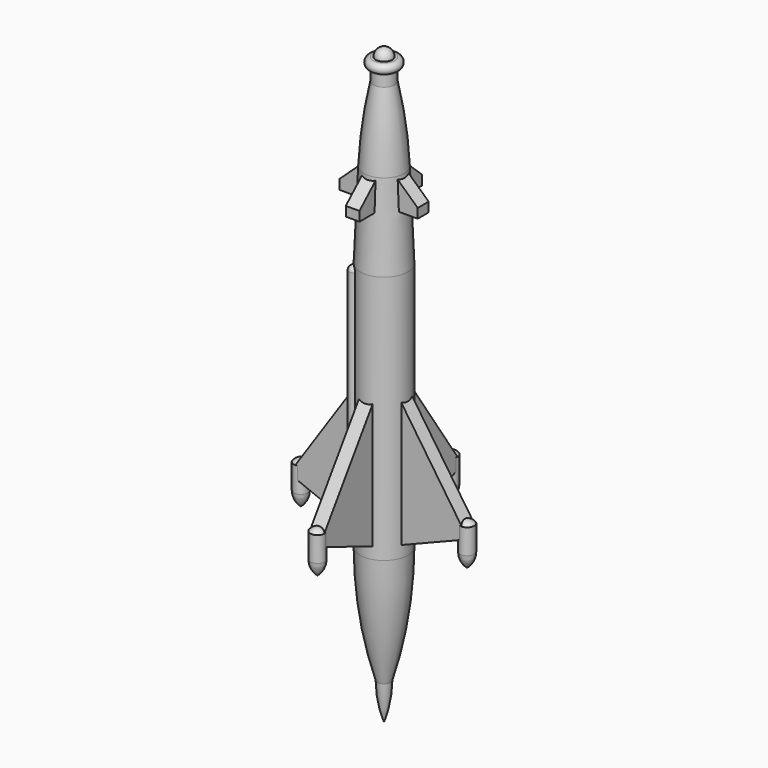
from build123d import *

# Parameters (mm, degrees)
F4_DEPTH     = 0.2
F7_COUNT     = 4
F10_DEPTH    = 6.25
F11_T4_ANGLE = 107.9477893391
F11_S5_R     = 0.1388888889
F11_T6_DEPTH = 2
F12_R        = 0.138879


# Not quite as in the source:
# - a fillet or chamfer that OpenCascade refuses, or shapes differently, is made with other operations: its cross-section is extruded or revolved along the edge and cut away or added
# - a fillet or chamfer is up to 0.001 mm smaller than in the source, because OpenCascade refuses the exact size
# - a feature names something its author has since deleted; it is built from what else it names


with BuildPart() as f2:
    # F1 (on Front) → F2 (revolve)
    with BuildSketch(Plane.XZ):
        with BuildLine():
            Line((0, 17.3611111111), (0, 0))
            ThreePointArc((0, 0), (0.1428592565, 0.5297895315), (0.1909722222, 1.0763888889))
            ThreePointArc((0.1909722222, 1.0763888889), (0.5679085065, 2.7768014898), (0.6944444444, 4.5138888889))
            Line((0.6944444444, 4.5138888889), (0.6944444444, 11.8055555556))
            Line((0.6944444444, 11.8055555556), (0.5902777778, 14.3055555556))
            ThreePointArc((0.5902777778, 14.3055555556), (0.4977180332, 15.4051886215), (0.3125, 16.4930555556))
            Line((0.3125, 16.4930555556), (0.3125, 16.8402777778))
            ThreePointArc((0.3125, 16.8402777778), (0.4513888889, 16.9791666667), (0.3125, 17.1180555556))
            Line((0.3125, 17.1180555556), (0.2430555556, 17.1180555556))
            ThreePointArc((0.2430555556, 17.1180555556), (0.1718662315, 17.2899217871), (0, 17.3611111111))
        make_face()
    revolve(axis=Axis((0, 0, 8.6805555556), (0, 0, 1)))

    # F3 (on Front) → F4 (join, symmetric)
    with BuildSketch(Plane.XZ):
        Polygon((0, 14.7382478632), (0, 4.5833333333), (2.4305555556, 5.5555555556), (2.4305555556, 5.9027777778), (0.4, 8.908), (0.4, 13.4027777778), (1.1458333333, 13.4027777778), (1.1458333333, 13.6805555556), align=None)
    extrude(amount=F4_DEPTH, both=True)

    # F5 (on Front) → F6 (revolve)
    with BuildSketch(Plane.XZ):
        with BuildLine():
            Line((2.4305555556, 5.9027777778), (2.4305555556, 4.7569444444))
            ThreePointArc((2.4305555556, 4.7569444444), (2.5839030509, 4.9406873635), (2.6388888889, 5.1736111111))
            Line((2.6388888889, 5.1736111111), (2.6388888889, 5.9027777778))
            ThreePointArc((2.6388888889, 5.9027777778), (2.5470174294, 5.9794515254), (2.4305555556, 6.0069444444))
            Line((2.4305555556, 6.0069444444), (2.4305555556, 5.9027777778))
        make_face()
    revolve(axis=Axis((2.4305555556, 0, 5.3819444444), (0, 0, 1)))

    # F7: F2 ×4 about axis
    f7_axis = Axis((0, 0, 4.5138888889), (0, 0, 1))


with BuildPart() as f2_1:
    add(f2.part)
    for i in range(1, F7_COUNT):
        add(f2.part.rotate(f7_axis, i * 360 / F7_COUNT))

    # F9 (on offset) → F10 (join)
    with BuildSketch(Plane.XY.offset(5.5555555556)):
        with BuildLine():
            Line((-0.3928371007, -0.589255651), (-0.0580600084, -0.2544785587))
            Line((-0.0580600084, -0.2544785587), (-0.2544785587, -0.0580600084))
            Line((-0.2544785587, -0.0580600084), (-0.589255651, -0.3928371007))
            ThreePointArc((-0.589255651, -0.3928371007), (-0.589255651, -0.589255651), (-0.3928371007, -0.589255651))
        make_face()
    extrude(amount=F10_DEPTH)

    # F11: chamfer of 0.2 on 1 edges, made by hand


with BuildPart() as f11_tool2:
    # F11_s3 → F11_t4 (revolve)
    with BuildSketch(Plane(origin=(0, 0, 0), x_dir=(0, 0, 1), z_dir=(0.1559844343, 0.9877595134, 0))):
        with BuildLine():
            Line((5.3498987013, -0.6887875902), (5.5612124098, -0.9001012987))
            Line((5.5612124098, -0.9001012987), (5.5652124098, -0.9001012987))
            ThreePointArc((5.5652124098, -0.9001012987), (5.5595555556, -0.7972728716), (5.5595555556, -0.6944444444))
            Line((5.5595555556, -0.6944444444), (5.5555555556, -0.6904444444))
            ThreePointArc((5.5555555556, -0.6904444444), (5.4527271284, -0.6904444444), (5.3498987013, -0.6847875902))
            Line((5.3498987013, -0.6847875902), (5.3498987013, -0.6887875902))
        make_face()
    revolve(axis=Axis((0, 0, 5.5555555556), (0, 0, 1)), revolution_arc=F11_T4_ANGLE)

    # F11_s5 → F11_t6 (intersect, symmetric)
    with BuildSketch(Plane.XY.offset(5.5)):
        with Locations((-0.4910463758, -0.4910463758)):
            Circle(F11_S5_R)
    extrude(amount=F11_T6_DEPTH, both=True, mode=Mode.INTERSECT)


with BuildPart() as f2_2:
    add(f2_1.part)

    # F11_t1: union F11_tool2
    add(f11_tool2.part)

    # F12 (radius 0.1388888889 in the source; OpenCascade refuses exactly that, so slightly less here)
    f12_edges = [f2_2.edges().sort_by_distance(p)[0] for p in [
        (-0.589256, -0.589256, 11.805556),
    ]]
    fillet(f12_edges, radius=F12_R)


solid = f2_2.part
